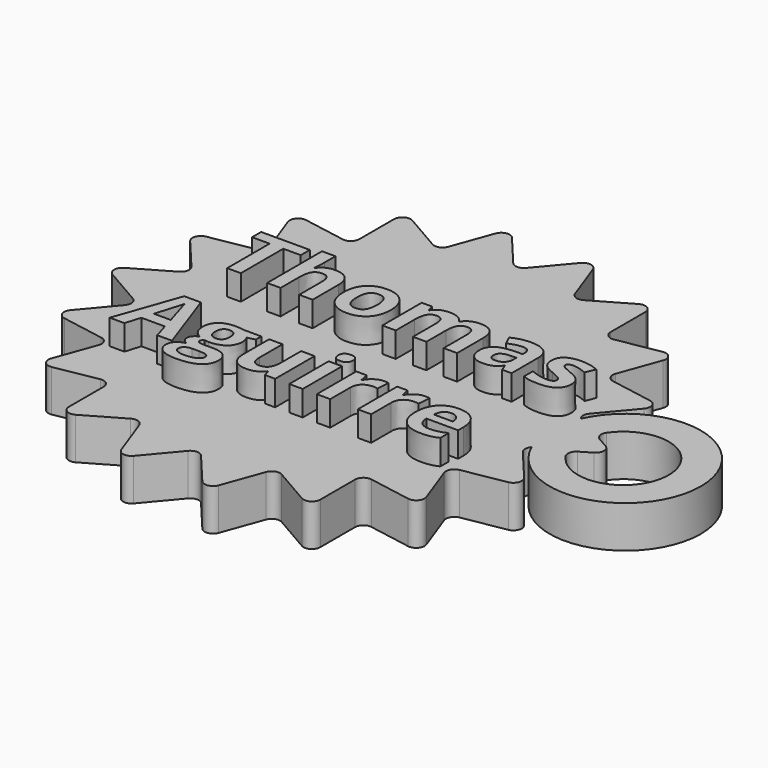
from build123d import *

# Parameters (mm, degrees)
F1_DEPTH      = 5
F2_R          = 1
F3_R          = 1
F4_R          = 9.02426598
F5_DEPTH      = 5
F7_DEPTH      = 5
F8_R          = 1
F10_DEPTH     = 4.5
F11_R         = 7.0893465871
F11_R_2       = 5.3736476411
F12_DEPTH     = 4.5
F13_TEXT_SIZE = 10.7679365461
F14_DEPTH     = 3


# Not quite as in the source:
# - a feature names something its author has since deleted; it is built from what else it names
# - Text() gives the source's letters only with a copy of the font that has no kerning and outlines rounded to 1/6400 em; it was checked with that copy


with BuildPart() as f1:
    # F0 (on Top) → F1 (new body)
    with BuildSketch(Plane.XY):
        Polygon((-69.4327632519, 10.2606042998), (-64.2233179219, 4.0522291123), (-71.2419846284, 0), (-64.2233179219, -4.0522291123), (-69.4327632519, -10.2606042998), (-61.4514299584, -11.6679287015), (-64.2233179219, -19.2836282906), (-56.2419846284, -17.8763038889), (-56.2419846284, -25.9807621135), (-49.2233179219, -21.9285330012), (-46.4514299584, -29.5442325904), (-41.2419846284, -23.3358574029), (-36.0325392983, -29.5442325904), (-33.2606513348, -21.9285330012), (-26.2419846284, -25.9807621135), (-26.2419846284, -17.8763038889), (-18.2606513348, -19.2836282906), (-21.0325392984, -11.6679287015), (-13.0512060048, -10.2606042998), (-18.2606513348, -4.0522291123), (-11.2419846284, 0), (-18.2606513348, 4.0522291123), (-13.0512060048, 10.2606042998), (-21.0325392984, 11.6679287015), (-18.2606513348, 19.2836282906), (-26.2419846284, 17.8763038889), (-26.2419846284, 25.9807621135), (-33.2606513348, 21.9285330012), (-36.0325392984, 29.5442325904), (-41.2419846284, 23.3358574029), (-46.4514299584, 29.5442325904), (-49.2233179219, 21.9285330012), (-56.2419846284, 25.9807621135), (-56.2419846284, 17.8763038889), (-64.2233179219, 19.2836282906), (-61.4514299584, 11.6679287015), align=None)
    extrude(amount=F1_DEPTH)

    # F2
    f2_edges = [f1.edges().sort_by_distance(p)[0] for p in [
        (-49.223318, -21.928533, 2.5),
        (-56.241985, -17.876304, 2.5),
        (-61.45143, -11.667929, 2.5),
        (-64.223318, -4.052229, 2.5),
        (-64.223318, 4.052229, 2.5),
        (-61.45143, 11.667929, 2.5),
        (-56.241985, 17.876304, 2.5),
        (-49.223318, 21.928533, 2.5),
        (-41.241985, 23.335857, 2.5),
        (-33.260651, 21.928533, 2.5),
        (-41.241985, -23.335857, 2.5),
        (-33.260651, -21.928533, 2.5),
        (-26.241985, -17.876304, 2.5),
        (-21.032539, -11.667929, 2.5),
        (-26.241985, 17.876304, 2.5),
        (-21.032539, 11.667929, 2.5),
        (-18.260651, 4.052229, 2.5),
        (-18.260651, -4.052229, 2.5),
    ]]
    fillet(f2_edges, radius=F2_R)

    # F3
    f3_edges = [f1.edges().sort_by_distance(p)[0] for p in [
        (-36.032539, 29.544233, 2.5),
        (-26.241985, 25.980762, 2.5),
        (-18.260651, 19.283628, 2.5),
        (-13.051206, 10.260604, 2.5),
        (-11.241985, 0, 2.5),
        (-13.051206, -10.260604, 2.5),
        (-56.241985, 25.980762, 2.5),
        (-46.45143, 29.544233, 2.5),
        (-64.223318, 19.283628, 2.5),
        (-69.432763, 10.260604, 2.5),
        (-71.241985, 0, 2.5),
        (-69.432763, -10.260604, 2.5),
        (-64.223318, -19.283628, 2.5),
        (-56.241985, -25.980762, 2.5),
        (-46.45143, -29.544233, 2.5),
        (-36.032539, -29.544233, 2.5),
        (-26.241985, -25.980762, 2.5),
        (-18.260651, -19.283628, 2.5),
    ]]
    fillet(f3_edges, radius=F3_R)

    # F4 (on Top) → F5 (join, through all)
    with BuildSketch(Plane.XY):
        with Locations((-9.2419846284, 0)):
            Circle(F4_R)
    extrude(amount=F5_DEPTH)

    # F6 (on face) → F7 (cut, through all)
    with BuildSketch(Plane.XY.offset(5)):
        with BuildLine():
            ThreePointArc((-14.3705448136, -2.1852792706), (-3.981082649, -0.0942598595), (-14.3705448136, 1.9967595517))
            Line((-14.3705448136, 1.9967595517), (-10.7515631244, 0))
            Line((-10.7515631244, 0), (-14.3705448136, -2.1852792706))
        make_face()
    extrude(amount=-F7_DEPTH, mode=Mode.SUBTRACT)

    # F8
    f8_edges = [f1.edges().sort_by_distance(p)[0] for p in [
        (-10.751563, 0, 2.5),
        (-14.370545, -2.185279, 2.5),
        (-14.370545, 1.99676, 2.5),
    ]]
    fillet(f8_edges, radius=F8_R)

    # F9 (on face) → F10 (cut)
    with BuildSketch(Plane.XY):
        with BuildLine():
            ThreePointArc((-35.3777156799, -4.6599307489), (-35.5753046169, -4.908160303), (-35.7829730175, -5.1480209603))
            Line((-35.7829730175, -5.1480209603), (-21.9766725259, -17.609254409))
            Line((-21.9766725259, -17.609254409), (-20.5904544794, -15.9396992978))
            Line((-20.5904544794, -15.9396992978), (-35.3777156799, -4.6599307489))
        make_face()
        with BuildLine():
            Line((-35.0430152336, -4.1849240607), (-22.1269458204, -12.5734481191))
            Line((-22.1269458204, -12.5734481191), (-20.8090839907, -10.2629405882))
            Line((-20.8090839907, -10.2629405882), (-34.6043804511, -3.4158988524))
            ThreePointArc((-34.6043804511, -3.4158988524), (-34.8126121734, -3.8067344742), (-35.0430152336, -4.1849240607))
        make_face()
        with BuildLine():
            ThreePointArc((-34.1823081919, -2.3833949122), (-34.2698744439, -2.6366901562), (-34.3662212872, -2.8867773708))
            Line((-34.3662212872, -2.8867773708), (-17.1305497448, -9.8744736155))
            Line((-17.1305497448, -9.8744736155), (-16.3989523541, -7.8314905025))
            Line((-16.3989523541, -7.8314905025), (-19.4509472573, -6.8787666419))
            Line((-19.4509472573, -6.8787666419), (-34.1823081919, -2.3833949122))
        make_face()
        with BuildLine():
            Line((-34.0002869576, -1.7286818538), (-18.9941076397, -5.1937600989))
            Line((-18.9941076397, -5.1937600989), (-18.54596272, -2.5718579299))
            Line((-18.54596272, -2.5718579299), (-33.8511272013, -0.8560126092))
            ThreePointArc((-33.8511272013, -0.8560126092), (-33.9131273587, -1.2944974025), (-34.0002869576, -1.7286818538))
        make_face()
        with BuildLine():
            ThreePointArc((-33.8115942061, 0.3570473634), (-33.8033972316, 0.0398847724), (-33.8083009973, -0.2773458261))
            Line((-33.8083009973, -0.2773458261), (-15.2221347635, -0.9486855723))
            Line((-15.2221347635, -0.9486855723), (-15.2333994712, 1.2213116278))
            Line((-15.2333994712, 1.2213116278), (-33.8115942061, 0.3570473634))
        make_face()
        with BuildLine():
            Line((-33.8605272028, 0.9360648973), (-18.5742046736, 2.812372041))
            Line((-18.5742046736, 2.812372041), (-19.0498295551, 5.4294287513))
            Line((-19.0498295551, 5.4294287513), (-34.0188333405, 1.807121388))
            ThreePointArc((-34.0188333405, 1.807121388), (-33.9271237992, 1.3738751607), (-33.8605272028, 0.9360648973))
        make_face()
        with BuildLine():
            ThreePointArc((-34.3965754224, 2.9605459736), (-34.2803967911, 2.6653141576), (-34.1765055688, 2.3655377184))
            Line((-34.1765055688, 2.3655377184), (-16.481610594, 8.0915279521))
            Line((-16.481610594, 8.0915279521), (-17.2343787101, 10.1268055511))
            Line((-17.2343787101, 10.1268055511), (-34.3965754224, 2.9605459736))
        make_face()
        with BuildLine():
            Line((-34.6405930582, 3.4879084069), (-20.9178834168, 10.4792906065))
            Line((-20.9178834168, 10.4792906065), (-22.2599107194, 12.7758461952))
            Line((-22.2599107194, 12.7758461952), (-35.0872710335, 4.2522898756))
            ThreePointArc((-35.0872710335, 4.2522898756), (-34.8529133175, 3.8765381033), (-34.6405930582, 3.4879084069))
        make_face()
        with BuildLine():
            ThreePointArc((-35.8367269225, 5.2069590463), (-35.6265794919, 4.9692673195), (-35.4264240963, 4.7231025025))
            Line((-35.4264240963, 4.7231025025), (-20.7570658633, 16.1557837872))
            Line((-20.7570658633, 16.1557837872), (-22.1605424433, 17.8108572693))
            Line((-22.1605424433, 17.8108572693), (-35.8367269225, 5.2069590463))
        make_face()
        with BuildLine():
            Line((-36.2463970692, 5.6190586866), (-25.742461624, 16.882252067))
            Line((-25.742461624, 16.882252067), (-27.7890230487, 18.5813080366))
            Line((-27.7890230487, 18.5813080366), (-36.927570926, 6.184569447))
            ThreePointArc((-36.927570926, 6.184569447), (-36.5788320346, 5.911633339), (-36.2463970692, 5.6190586866))
        make_face()
        with BuildLine():
            ThreePointArc((-37.958345181, 6.8253360115), (-37.6795758328, 6.6738535042), (-37.4072979585, 6.5109914192))
            Line((-37.4072979585, 6.5109914192), (-27.5328175668, 22.2714136636))
            Line((-27.5328175668, 22.2714136636), (-29.4177226221, 23.3466567405))
            Line((-29.4177226221, 23.3466567405), (-37.958345181, 6.8253360115))
        make_face()
        with BuildLine():
            Line((-38.4842555729, 7.0724675602), (-32.4660239601, 21.2489647728))
            Line((-32.4660239601, 21.2489647728), (-34.9702739951, 22.1455898979))
            Line((-34.9702739951, 22.1455898979), (-39.3177656909, 7.3708986687))
            ThreePointArc((-39.3177656909, 7.3708986687), (-38.8967086813, 7.2336983476), (-38.4842555729, 7.0724675602))
        make_face()
        with BuildLine():
            ThreePointArc((-40.5055317243, 7.6204767225), (-40.191764156, 7.5734744606), (-39.8802045331, 7.5135586787))
            Line((-39.8802045331, 7.5135586787), (-35.9916100498, 25.7007823611))
            Line((-35.9916100498, 25.7007823611), (-38.1305962124, 26.0665048489))
            Line((-38.1305962124, 26.0665048489), (-40.5055317243, 7.6204767225))
        make_face()
        with BuildLine():
            Line((-41.0842498064, 7.6728324676), (-40.2776095782, 23.0527387256))
            Line((-40.2776095782, 23.0527387256), (-42.9374987105, 23.0387867834))
            Line((-42.9374987105, 23.0387867834), (-41.9695625642, 7.668188728))
            ThreePointArc((-41.9695625642, 7.668188728), (-41.5269731258, 7.6832725775), (-41.0842498064, 7.6728324676))
        make_face()
        with BuildLine():
            ThreePointArc((-43.1710582627, 7.4964754745), (-42.8601374738, 7.5596226245), (-42.5468747909, 7.6098798733))
            Line((-42.5468747909, 7.6098798733), (-45.1131881003, 26.0302574027))
            Line((-45.1131881003, 26.0302574027), (-47.2482620709, 25.6423477718))
            Line((-47.2482620709, 25.6423477718), (-43.1710582627, 7.4964754745))
        make_face()
        with BuildLine():
            Line((-43.7327820934, 7.3477405404), (-48.235025966, 22.0760121659))
            Line((-48.235025966, 22.0760121659), (-50.7297323105, 21.1531659665))
            Line((-50.7297323105, 21.1531659665), (-44.5631157065, 7.0405820563))
            ThreePointArc((-44.5631157065, 7.0405820563), (-44.1523766576, 7.2061307415), (-43.7327820934, 7.3477405404))
        make_face()
        with BuildLine():
            ThreePointArc((-45.6334229567, 6.468288648), (-45.362850583, 6.6339687317), (-45.085668943, 6.7883372453))
            Line((-45.085668943, 6.7883372453), (-53.7973547852, 23.2200992358))
            Line((-53.7973547852, 23.2200992358), (-55.6709951327, 22.1253451128))
            Line((-55.6709951327, 22.1253451128), (-45.6334229567, 6.468288648))
        make_face()
        with BuildLine():
            Line((-46.1104003519, 6.1364026629), (-55.3784912683, 18.4365927318))
            Line((-55.3784912683, 18.4365927318), (-57.4071164218, 16.7161611466))
            Line((-57.4071164218, 16.7161611466), (-46.7856043321, 5.5637772807))
            ThreePointArc((-46.7856043321, 5.5637772807), (-46.4562568639, 5.8598231869), (-46.1104003519, 6.1364026629))
        make_face()
        with BuildLine():
            ThreePointArc((-47.5956282836, 4.6599307489), (-47.3980393467, 4.908160303), (-47.190370946, 5.1480209603))
            Line((-47.190370946, 5.1480209603), (-60.9966714376, 17.609254409))
            Line((-60.9966714376, 17.609254409), (-62.3828894841, 15.9396992978))
            Line((-62.3828894841, 15.9396992978), (-47.5956282836, 4.6599307489))
        make_face()
        with BuildLine():
            Line((-47.93032873, 4.1849240607), (-60.8463981431, 12.5734481191))
            Line((-60.8463981431, 12.5734481191), (-62.1642599729, 10.2629405882))
            Line((-62.1642599729, 10.2629405882), (-48.3689635124, 3.4158988524))
            ThreePointArc((-48.3689635124, 3.4158988524), (-48.1607317901, 3.8067344742), (-47.93032873, 4.1849240607))
        make_face()
        with BuildLine():
            ThreePointArc((-48.821003322, 2.2895164282), (-48.7202299636, 2.590355305), (-48.6071226764, 2.8867773708))
            Line((-48.6071226764, 2.8867773708), (-65.8427942188, 9.8744736155))
            Line((-65.8427942188, 9.8744736155), (-66.5743916094, 7.8314905025))
            Line((-66.5743916094, 7.8314905025), (-48.821003322, 2.2895164282))
        make_face()
        with BuildLine():
            Line((-48.973057006, 1.7286818538), (-63.9792363238, 5.1937600989))
            Line((-63.9792363238, 5.1937600989), (-64.4273812436, 2.5718579299))
            Line((-64.4273812436, 2.5718579299), (-49.1222167623, 0.8560126092))
            ThreePointArc((-49.1222167623, 0.8560126092), (-49.0602166048, 1.2944974025), (-48.973057006, 1.7286818538))
        make_face()
        Polygon((-49.1617497575, -0.3570473634), (-49.1650429663, 0.2773458261), (-67.7512092001, 0.9486855723), (-67.7399444924, -1.2213116278), align=None)
        with BuildLine():
            ThreePointArc((-48.5767685411, -2.9605459736), (-48.6929471725, -2.6653141576), (-48.7968383947, -2.3655377184))
            Line((-48.7968383947, -2.3655377184), (-66.4917333696, -8.0915279521))
            Line((-66.4917333696, -8.0915279521), (-65.7389652535, -10.1268055511))
            Line((-65.7389652535, -10.1268055511), (-48.5767685411, -2.9605459736))
        make_face()
        with BuildLine():
            Line((-49.1128167608, -0.9360648973), (-64.39913929, -2.812372041))
            Line((-64.39913929, -2.812372041), (-63.9235144085, -5.4294287513))
            Line((-63.9235144085, -5.4294287513), (-48.954510623, -1.807121388))
            ThreePointArc((-48.954510623, -1.807121388), (-49.0462201644, -1.3738751607), (-49.1128167608, -0.9360648973))
        make_face()
        with BuildLine():
            Line((-48.3327509053, -3.4879084069), (-62.0554605467, -10.4792906065))
            Line((-62.0554605467, -10.4792906065), (-60.7134332442, -12.7758461952))
            Line((-60.7134332442, -12.7758461952), (-47.88607293, -4.2522898756))
            ThreePointArc((-47.88607293, -4.2522898756), (-48.1204306461, -3.8765381033), (-48.3327509053, -3.4879084069))
        make_face()
        with BuildLine():
            ThreePointArc((-47.1366170411, -5.2069590463), (-47.3467644716, -4.9692673195), (-47.5469198672, -4.7231025025))
            Line((-47.5469198672, -4.7231025025), (-62.2162781003, -16.1557837872))
            Line((-62.2162781003, -16.1557837872), (-60.8128015203, -17.8108572693))
            Line((-60.8128015203, -17.8108572693), (-47.1366170411, -5.2069590463))
        make_face()
        with BuildLine():
            Line((-46.7269468943, -5.6190586866), (-57.2308823396, -16.882252067))
            Line((-57.2308823396, -16.882252067), (-55.1843209149, -18.5813080366))
            Line((-55.1843209149, -18.5813080366), (-46.0457730376, -6.184569447))
            ThreePointArc((-46.0457730376, -6.184569447), (-46.394511929, -5.911633339), (-46.7269468943, -5.6190586866))
        make_face()
        with BuildLine():
            ThreePointArc((-45.0149987825, -6.8253360115), (-45.2937681308, -6.6738535042), (-45.566046005, -6.5109914192))
            Line((-45.566046005, -6.5109914192), (-55.4405263967, -22.2714136636))
            Line((-55.4405263967, -22.2714136636), (-53.5556213415, -23.3466567405))
            Line((-53.5556213415, -23.3466567405), (-45.0149987825, -6.8253360115))
        make_face()
        with BuildLine():
            Line((-44.4890883907, -7.0724675602), (-50.5073200035, -21.2489647728))
            Line((-50.5073200035, -21.2489647728), (-48.0030699685, -22.1455898979))
            Line((-48.0030699685, -22.1455898979), (-43.6555782727, -7.3708986687))
            ThreePointArc((-43.6555782727, -7.3708986687), (-44.0766352823, -7.2336983476), (-44.4890883907, -7.0724675602))
        make_face()
        with BuildLine():
            ThreePointArc((-42.4678122393, -7.6204767225), (-42.7815798076, -7.5734744606), (-43.0931394305, -7.5135586787))
            Line((-43.0931394305, -7.5135586787), (-46.9817339137, -25.7007823611))
            Line((-46.9817339137, -25.7007823611), (-44.8427477512, -26.0665048489))
            Line((-44.8427477512, -26.0665048489), (-42.4678122393, -7.6204767225))
        make_face()
        with BuildLine():
            Line((-41.8890941571, -7.6728324676), (-42.6957343854, -23.0527387256))
            Line((-42.6957343854, -23.0527387256), (-40.0358452531, -23.0387867834))
            Line((-40.0358452531, -23.0387867834), (-41.0037813994, -7.668188728))
            ThreePointArc((-41.0037813994, -7.668188728), (-41.4463708377, -7.6832725775), (-41.8890941571, -7.6728324676))
        make_face()
        with BuildLine():
            ThreePointArc((-39.8022857009, -7.4964754745), (-40.1132064898, -7.5596226245), (-40.4264691727, -7.6098798733))
            Line((-40.4264691727, -7.6098798733), (-37.8601558633, -26.0302574027))
            Line((-37.8601558633, -26.0302574027), (-35.7250818926, -25.6423477718))
            Line((-35.7250818926, -25.6423477718), (-39.8022857009, -7.4964754745))
        make_face()
        with BuildLine():
            Line((-39.2405618701, -7.3477405404), (-34.7383179975, -22.0760121659))
            Line((-34.7383179975, -22.0760121659), (-32.2436116531, -21.1531659665))
            Line((-32.2436116531, -21.1531659665), (-38.4102282571, -7.0405820563))
            ThreePointArc((-38.4102282571, -7.0405820563), (-38.8209673059, -7.2061307415), (-39.2405618701, -7.3477405404))
        make_face()
        with BuildLine():
            ThreePointArc((-37.3399210068, -6.468288648), (-37.6104933805, -6.6339687317), (-37.8876750206, -6.7883372453))
            Line((-37.8876750206, -6.7883372453), (-29.1759891784, -23.2200992358))
            Line((-29.1759891784, -23.2200992358), (-27.3023488309, -22.1253451128))
            Line((-27.3023488309, -22.1253451128), (-37.3399210068, -6.468288648))
        make_face()
        with BuildLine():
            Line((-36.8629436116, -6.1364026629), (-27.5948526953, -18.4365927318))
            Line((-27.5948526953, -18.4365927318), (-25.5662275418, -16.7161611466))
            Line((-25.5662275418, -16.7161611466), (-36.1877396314, -5.5637772807))
            ThreePointArc((-36.1877396314, -5.5637772807), (-36.5170870997, -5.8598231869), (-36.8629436116, -6.1364026629))
        make_face()
    extrude(amount=F10_DEPTH, mode=Mode.SUBTRACT)

    # F11 (on face) → F12 (cut, through all)
    with BuildSketch(Plane.XY):
        with Locations((-41.4866719818, 0)):
            Circle(F11_R)
        with Locations((-41.4866719818, 0)):
            Circle(F11_R_2, mode=Mode.SUBTRACT)
    extrude(amount=F12_DEPTH, mode=Mode.SUBTRACT)

    # F13 (on face) → F14 (join)
    with BuildSketch(Plane.XY.offset(5)):
        with Locations((-60.908870383, 2.3123007417)):
            Text('Thomas', F13_TEXT_SIZE, font='Open Sans', font_style=FontStyle.BOLD, text_align=(TextAlign.LEFT, TextAlign.BOTTOM))
        with Locations((-60.908870383, -12.332092961)):
            Text('Aguirre', F13_TEXT_SIZE, font='Open Sans', font_style=FontStyle.BOLD, text_align=(TextAlign.LEFT, TextAlign.BOTTOM))
    extrude(amount=F14_DEPTH)


solid = f1.part
